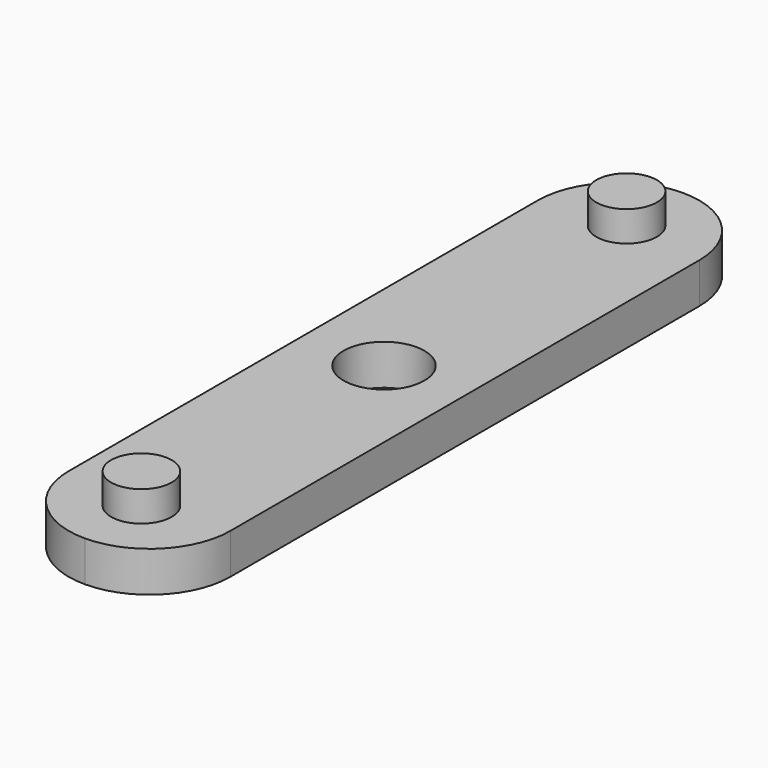
from build123d import *

# Parameters (mm, degrees)
F0_W     = 8
F0_H     = 37
F0_R     = 2
F1_DEPTH = 2
F2_R     = 1.5
F3_DEPTH = 1.5
F4_R     = 3.99999


# Not quite as in the source:
# - a fillet or chamfer is up to 0.001 mm smaller than in the source, because OpenCascade refuses the exact size


with BuildPart() as f1:
    # F0 (on Top) → F1 (new body)
    with BuildSketch(Plane.XY):
        Rectangle(F0_W, F0_H)
        Circle(F0_R, mode=Mode.SUBTRACT)
    extrude(amount=F1_DEPTH)

    # F2 (on face) → F3 (join)
    with BuildSketch(Plane.XY.offset(2)):
        with Locations((0, 15)):
            Circle(F2_R)
        with Locations((0, -15)):
            Circle(F2_R)
    extrude(amount=F3_DEPTH)

    # F4 (radius 4 in the source; OpenCascade refuses exactly that, so slightly less here)
    f4_edges = [f1.edges().sort_by_distance(p)[0] for p in [
        (-4, 18.5, 1),
        (4, 18.5, 1),
        (4, -18.5, 1),
        (-4, -18.5, 1),
    ]]
    fillet(f4_edges, radius=F4_R)


solid = f1.part
